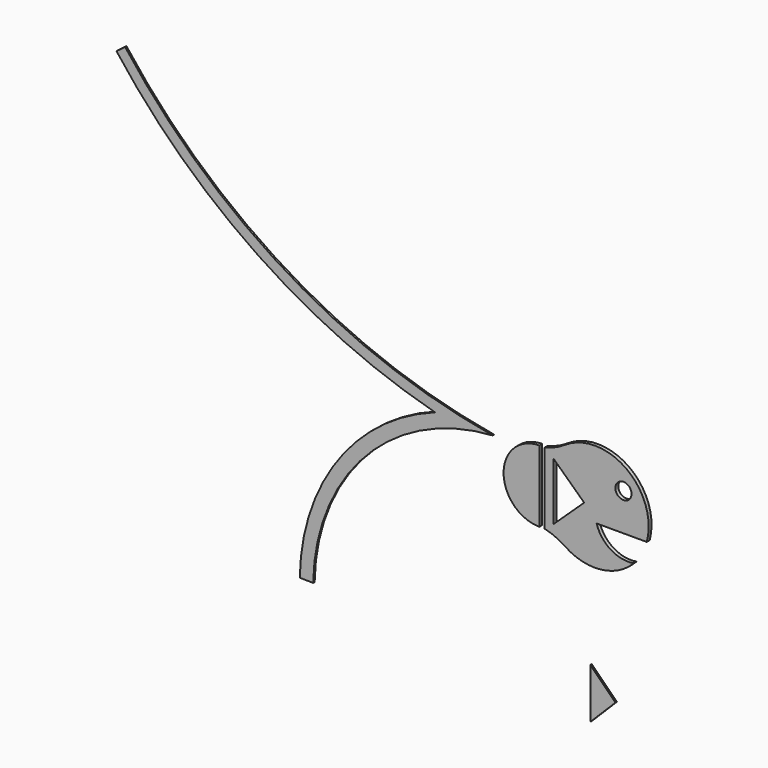
from build123d import *

# Parameters (mm, degrees)
F5_R     = 4.5
F6_DEPTH = 2
F8_DEPTH = 1
F9_DEPTH = 1


# Not quite as in the source:
# - a feature names something its author has since deleted; it is built from what else it names


with BuildPart() as f6:
    # F5 (on offset) → F6 (new body)
    with BuildSketch(Plane.XZ.offset(25)):
        with BuildLine():
            ThreePointArc((-398.467205436, -39.2777054383), (-392.6082274756, -41.2404384818), (-387.1915217022, -44.2135248081))
            ThreePointArc((-387.1915217022, -44.2135248081), (-367.2251337414, -49.1320591827), (-348.7819741916, -40.0381879271))
            ThreePointArc((-348.7819741916, -40.0381879271), (-361.6011790718, -37.5934442718), (-369.5320105339, -27.229531033))
            Line((-369.5320105339, -27.229531033), (-341.5320105339, -27.229531033))
            ThreePointArc((-341.5320105339, -27.229531033), (-352.9546885172, 5.0502340302), (-387.1915217022, 5.598009817))
            ThreePointArc((-387.1915217022, 5.598009817), (-392.6082274756, 2.6249234907), (-398.467205436, 0.6621904472))
            Line((-398.467205436, 0.6621904472), (-398.467205436, -39.2777054383))
        make_face()
        Polygon((-393.467205436, -3.3077574955), (-376.467205436, -19.3077574955), (-393.467205436, -35.3077574955), (-393.467205436, -19.3077574955), align=None, mode=Mode.SUBTRACT)
        with Locations((-354.5545938938, -6.4046481277)):
            Circle(F5_R, mode=Mode.SUBTRACT)
    extrude(amount=F6_DEPTH)


with BuildPart() as f6b:
    # F5 (on offset) → F6, piece 2 (new body)
    with BuildSketch(Plane.XZ.offset(25)):
        with BuildLine():
            Line((-401.467205436, -39.2777054383), (-401.467205436, 0.6621904472))
            ThreePointArc((-401.467205436, 0.6621904472), (-421.4371533787, -19.3077574955), (-401.467205436, -39.2777054383))
        make_face()
    extrude(amount=F6_DEPTH)


with BuildPart() as f8:
    # F7 (on Front) → F8 (new body)
    with BuildSketch(Plane.XZ):
        with BuildLine():
            Line((-653.4249486684, 103.9134022917), (-658.2025638487, 100.2837475989))
            ThreePointArc((-658.2025638487, 100.2837475989), (-579.2555377986, 25.744047787), (-480.467205436, -19.3077574955))
            ThreePointArc((-480.467205436, -19.3077574955), (-534.7020128056, -60.4384507793), (-555.9372290567, -125.1084890597))
            Line((-555.9372290567, -125.1084890597), (-548.4414986364, -125.2204015407))
            ThreePointArc((-548.4414986364, -125.2204015407), (-518.9281051059, -53.0898043717), (-448.2662559395, -20.2147907898))
            ThreePointArc((-448.2662559395, -20.2147907898), (-562.684901543, 22.2813486703), (-653.4249486684, 103.9134022917))
        make_face()
    extrude(amount=F8_DEPTH)

    # F7 (on Front) → F9 (join)
    with BuildSketch(Plane.XZ):
        with BuildLine():
            Line((-653.4249486684, 103.9134022917), (-658.2025638487, 100.2837475989))
            ThreePointArc((-658.2025638487, 100.2837475989), (-579.2555377986, 25.744047787), (-480.467205436, -19.3077574955))
            ThreePointArc((-480.467205436, -19.3077574955), (-534.7020128056, -60.4384507793), (-555.9372290567, -125.1084890597))
            Line((-555.9372290567, -125.1084890597), (-548.4414986364, -125.2204015407))
            ThreePointArc((-548.4414986364, -125.2204015407), (-518.9281051059, -53.0898043717), (-448.2662559395, -20.2147907898))
            ThreePointArc((-448.2662559395, -20.2147907898), (-562.684901543, 22.2813486703), (-653.4249486684, 103.9134022917))
        make_face()
    extrude(amount=F9_DEPTH)


with BuildPart() as f9:
    # F7 (on Front) → F9, piece 2 (new body)
    with BuildSketch(Plane.XZ):
        Polygon((-379.8274085522, -129.1934684515), (-393.8274085522, -115.1934684515), (-393.8274085522, -143.1934684515), align=None)
    extrude(amount=F9_DEPTH)


solid = Compound([f6.part, f6b.part, f8.part, f9.part])
